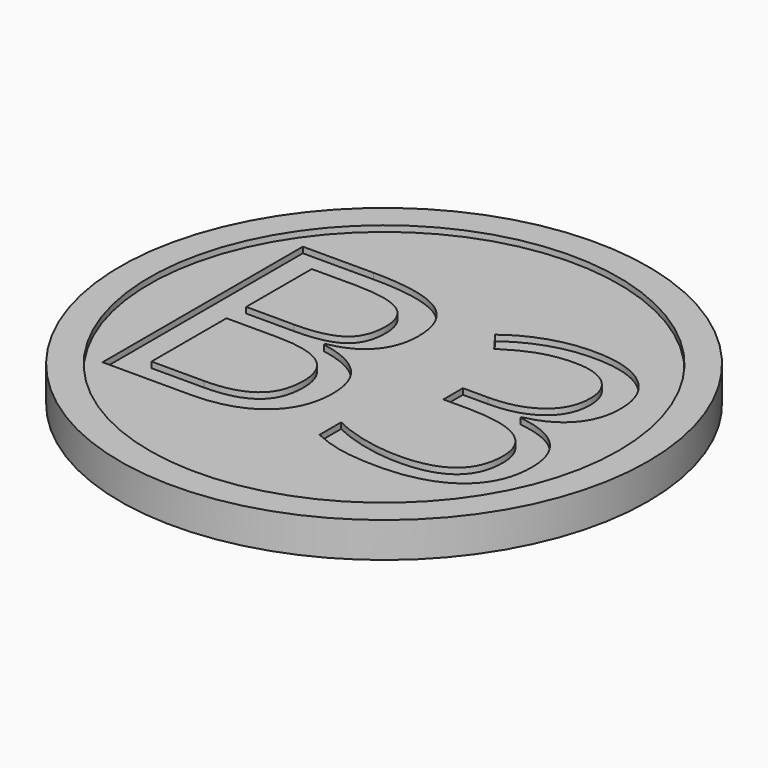
from build123d import *

# Parameters (mm, degrees)
F0_R          = 40
F1_DEPTH      = 2
F1_DEPTH_BACK = 2
F0_R_2        = 45
F2_DEPTH      = 3
F2_DEPTH_BACK = 3
F3_TEXT_SIZE  = 59.7862196403
F4_DEPTH      = 1


# Not quite as in the source:
# - Text() gives the source's letters only with a copy of the font that has no kerning and outlines rounded to 1/6400 em; it was checked with that copy


with BuildPart() as f1:
    # F0 (on Top) → F1 (new body, two sides)
    with BuildSketch(Plane.XY) as f1_sk:
        Circle(F0_R)
    extrude(amount=F1_DEPTH)
    extrude(f1_sk.sketch, amount=-F1_DEPTH_BACK)

    # F0 (on Top) → F2 (join, two sides)
    with BuildSketch(Plane.XY) as f2_sk:
        Circle(F0_R_2)
        Circle(F0_R, mode=Mode.SUBTRACT)
    extrude(amount=F2_DEPTH)
    extrude(f2_sk.sketch, amount=-F2_DEPTH_BACK)

    # F3 (on face) → F4 (cut)
    with BuildSketch(Plane.XY.offset(2)):
        with Locations((-36.6470843202, -21.5230390705)):
            Text('B3', F3_TEXT_SIZE, font='Open Sans', text_align=(TextAlign.LEFT, TextAlign.BOTTOM))
    extrude(amount=-F4_DEPTH, mode=Mode.SUBTRACT)


solid = f1.part
